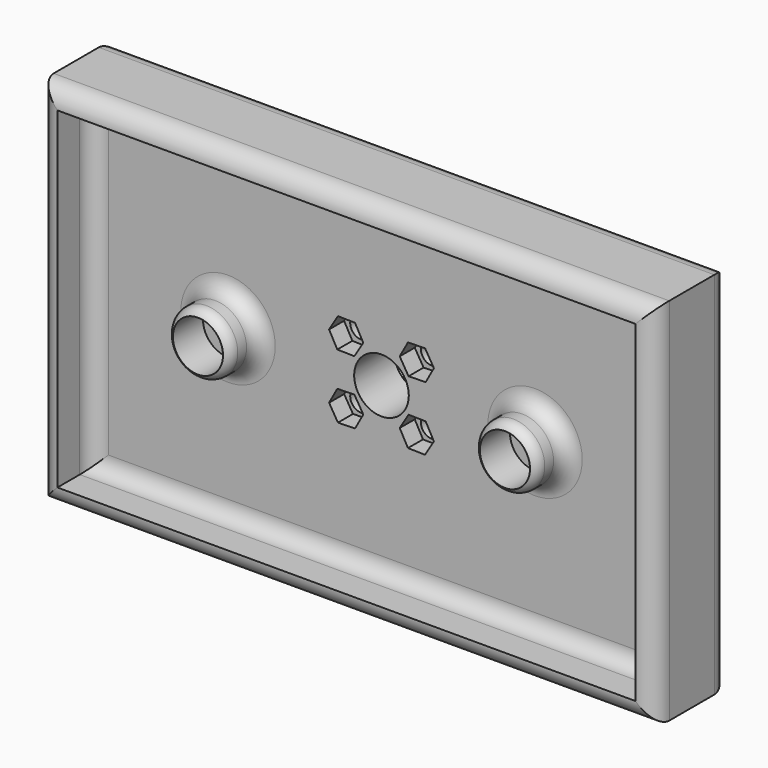
from build123d import *

# Parameters (mm, degrees)
F0_W     = 98.3085063696
F0_H     = 59.0165173113
F0_W_2   = 92.3085063696
F0_H_2   = 53.0165173113
F1_DEPTH = 8
F2_DEPTH = 15
F3_R     = 4.3592981544
F3_R_2   = 1.7500302992
F4_DEPTH = 8.001
F3_R_3   = 5
F3_R_4   = 4
F5_DEPTH = 6
F6_R     = 2.54
F7_R     = 1.7500302992
F8_DEPTH = 3
F9_R     = 3
F10_R    = 2.99999


# Not quite as in the source:
# - a fillet or chamfer that OpenCascade refuses, or shapes differently, is made with other operations: its cross-section is extruded or revolved along the edge and cut away or added
# - a fillet or chamfer is up to 0.001 mm smaller than in the source, because OpenCascade refuses the exact size


with BuildPart() as f1:
    # F0 (on Front) → F1 (new body)
    with BuildSketch(Plane.XZ):
        Rectangle(F0_W, F0_H)
        Rectangle(F0_W_2, F0_H_2, mode=Mode.SUBTRACT)
        Rectangle(F0_W_2, F0_H_2)
    extrude(amount=F1_DEPTH)

    # F0 (on Front) → F2 (join)
    with BuildSketch(Plane.XZ):
        Rectangle(F0_W, F0_H)
        Rectangle(F0_W_2, F0_H_2, mode=Mode.SUBTRACT)
    extrude(amount=F2_DEPTH)

    # F3 (on face) → F4 (cut, through all)
    with BuildSketch(Plane.XZ.offset(8)):
        Circle(F3_R)
        with Locations((5.6447647512, 5.1466971636)):
            Circle(F3_R_2)
        with Locations((-5.6447647512, 5.1466971636)):
            Circle(F3_R_2)
        with Locations((-5.6447647512, -5.1466971636)):
            Circle(F3_R_2)
        with Locations((5.6447647512, -5.1466971636)):
            Circle(F3_R_2)
    extrude(amount=-F4_DEPTH, mode=Mode.SUBTRACT)

    # F3 (on face) → F5 (join)
    with BuildSketch(Plane.XZ.offset(8)):
        with Locations((-24.5116613805, 0)):
            Circle(F3_R_3)
        with Locations((-24.5116613805, 0)):
            Circle(F3_R_4, mode=Mode.SUBTRACT)
        with Locations((24.5116613805, 0)):
            Circle(F3_R_3)
        with Locations((24.5116613805, 0)):
            Circle(F3_R_4, mode=Mode.SUBTRACT)
    extrude(amount=F5_DEPTH)

    # F6
    f6_edges = [f1.edges().sort_by_distance(p)[0] for p in [
        (-29.511661, -8, 0),
        (19.511661, -8, 0),
        (0, -8, -26.508259),
        (46.154253, -8, 0),
        (-46.154253, -8, 0),
        (0, -8, 26.508259),
    ]]
    fillet(f6_edges, radius=F6_R)

    # F7 (on face) → F8 (cut)
    with BuildSketch(Plane.XZ.offset(8)):
        Polygon((-2.9085768434, 5.0357150996), (-4.2244093493, 7.4292570353), (-6.9551937235, 7.4864836259), (-8.3701455918, 5.1501682809), (-7.054313086, 2.7566263452), (-4.3235287118, 2.6993997546), align=None)
        with Locations((-5.6447647512, 5.1466971636)):
            Circle(F7_R, mode=Mode.SUBTRACT)
        Polygon((8.3701455918, 5.1501682809), (6.9551937235, 7.4864836259), (4.2244093493, 7.4292570353), (2.9085768434, 5.0357150996), (4.3235287118, 2.6993997546), (7.054313086, 2.7566263452), align=None)
        with Locations((5.6447647512, 5.1466971636)):
            Circle(F7_R, mode=Mode.SUBTRACT)
        Polygon((4.3235287118, -2.6993997546), (2.9085768434, -5.0357150996), (4.2244093493, -7.4292570353), (6.9551937235, -7.4864836259), (8.3701455918, -5.1501682809), (7.054313086, -2.7566263452), align=None)
        with Locations((5.6447647512, -5.1466971636)):
            Circle(F7_R, mode=Mode.SUBTRACT)
        Polygon((-2.9085768434, -5.0357150996), (-4.3235287118, -2.6993997546), (-7.054313086, -2.7566263452), (-8.3701455918, -5.1501682809), (-6.9551937235, -7.4864836259), (-4.2244093493, -7.4292570353), align=None)
        with Locations((-5.6447647512, -5.1466971636)):
            Circle(F7_R, mode=Mode.SUBTRACT)
    extrude(amount=-F8_DEPTH, mode=Mode.SUBTRACT)

    # F9
    f9_edges = [f1.edges().sort_by_distance(p)[0] for p in [
        (0, 0, 29.508259),
        (49.154253, 0, 0),
        (0, 0, -29.508259),
        (-49.154253, 0, 0),
    ]]
    fillet(f9_edges, radius=F9_R)

    # F10 (radius 3 in the source; OpenCascade refuses exactly that, so slightly less here)
    f10_edges = [f1.edges().sort_by_distance(p)[0] for p in [
        (0, -15, -29.508259),
        (49.154253, -15, 0),
        (-49.154253, -15, 0),
        (0, -15, 29.508259),
    ]]
    fillet(f10_edges, radius=F10_R)

    # F11: fillet of radius 2 on 2 edges, made by hand

    # F11_s1 → F11_t2 (revolve, cut)
    with BuildSketch(Plane.XY):
        with BuildLine():
            ThreePointArc((29.5120613805, -12.2673917434), (29.2440686279, -13.2678330874), (28.5118614771, -14.0003463544))
            Line((28.5118614771, -14.0003463544), (28.6119780552, -14.1736418155))
            ThreePointArc((28.6119780552, -14.1736418155), (29.0117614288, -14.2001365685), (29.5116613805, -14.2001365685))
            Line((29.5116613805, -14.2001365685), (29.7117979491, -14))
            ThreePointArc((29.7117979491, -14), (29.7117979491, -13.1336958717), (29.7121979491, -12.2673917434))
            Line((29.7121979491, -12.2673917434), (29.5120613805, -12.2673917434))
        make_face()
    revolve(axis=Axis((24.5116613805, -14, 0), (0, -1, 0)), mode=Mode.SUBTRACT)

    # F11_s3 → F11_t4 (revolve, cut)
    with BuildSketch(Plane.XY):
        with BuildLine():
            ThreePointArc((-19.5112613805, -12.2673917434), (-19.7792541332, -13.2678330874), (-20.511461284, -14.0003463544))
            Line((-20.511461284, -14.0003463544), (-20.4113447058, -14.1736418155))
            ThreePointArc((-20.4113447058, -14.1736418155), (-20.0115613323, -14.2001365685), (-19.5116613805, -14.2001365685))
            Line((-19.5116613805, -14.2001365685), (-19.311524812, -14))
            ThreePointArc((-19.311524812, -14), (-19.311524812, -13.1336958717), (-19.311124812, -12.2673917434))
            Line((-19.311124812, -12.2673917434), (-19.5112613805, -12.2673917434))
        make_face()
    revolve(axis=Axis((-24.5116613805, -14, 0), (0, -1, 0)), mode=Mode.SUBTRACT)


solid = f1.part
